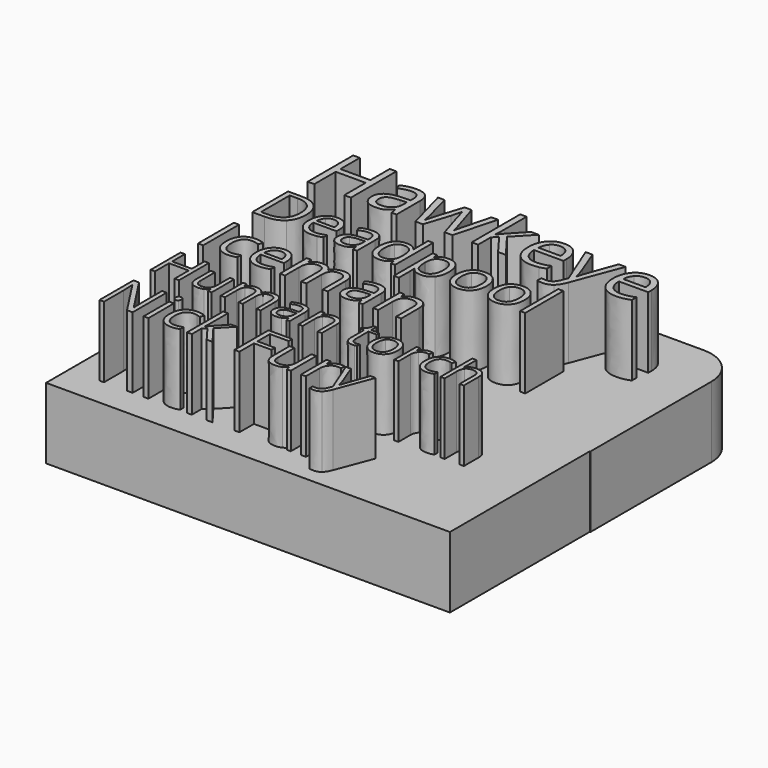
from build123d import *

# Parameters (mm, degrees)
F1_DEPTH     = 25.4
F3_DEPTH     = 25.4
F4_DEPTH     = 25.4
F5_DEPTH     = 25.4
F6_DEPTH     = 25.4
F2_W         = 1.8225440387
F2_H         = 17.0771322931
F7_DEPTH     = 25.4
F2_TEXT_SIZE = 22.4745314982
F8_DEPTH     = 25.4
F9_DEPTH     = 25.4
F10_DEPTH    = 25.4
F2_W_2       = 1.7290800267
F2_H_2       = 11.4105955517
F11_DEPTH    = 25.4
F12_DEPTH    = 25.4
F13_R        = 13.5243778387
F14_R        = 13.5128


# Not quite as in the source:
# - Text() gives the source's letters only with a copy of the font that has no kerning and outlines rounded to 1/6400 em; it was checked with that copy


with BuildPart() as f1:
    # F0 (on Top) → F1 (new body)
    with BuildSketch(Plane.XY):
        Polygon((72.1950531006, 67.6310360432), (-72.6100355387, 67.6310360432), (-72.6100355387, 0), (-72.6100355387, -62.6520514488), (71.9875991344, -62.6520514488), (71.9875991344, 0), (72.1950531006, 0), align=None)
    extrude(amount=F1_DEPTH)

    # F2 (on face) → F3 (join)
    with BuildSketch(Plane.XY.offset(25.4)):
        Polygon((-48.0028636327, 40.0392413139), (-45.6361505882, 40.0392413139), (-45.6361505882, 60.4036705045), (-48.0028636327, 60.4036705045), (-48.0028636327, 51.7390939349), (-58.7310713502, 51.7390939349), (-58.7310713502, 60.4036705045), (-61.0977843947, 60.4036705045), (-61.0977843947, 40.0392413139), (-58.7310713502, 40.0392413139), (-58.7310713502, 49.6219777463), (-48.0028636327, 49.6219777463), align=None)
        with BuildLine():
            Line((-31.4715290151, 42.2142996298), (-31.0124490837, 40.0392413139))
            Line((-31.0124490837, 40.0392413139), (-29.2964706993, 40.0392413139))
            Line((-29.2964706993, 40.0392413139), (-29.2964706993, 50.4599100483))
            add(Edge.make_bspline(
                [(-30.6135398229, 54.3442611185), (-29.2964706993, 53.134162076), (-29.2964706993, 50.4599100483)],
                knots=[0, 0, 0, 1, 1, 1], degree=2))
            add(Edge.make_bspline(
                [(-34.6583460147, 55.554360161), (-31.9306089465, 55.554360161), (-30.6135398229, 54.3442611185)],
                knots=[0, 0, 0, 1, 1, 1], degree=2))
            add(Edge.make_bspline(
                [(-37.3571120193, 55.2067073974), (-36.0133003754, 55.554360161), (-34.6583460147, 55.554360161)],
                knots=[0, 0, 0, 1, 1, 1], degree=2))
            add(Edge.make_bspline(
                [(-39.8285666015, 54.2484337542), (-38.7009236632, 54.8590546338), (-37.3571120193, 55.2067073974)],
                knots=[0, 0, 0, 1, 1, 1], degree=2))
            Line((-39.8285666015, 54.2484337542), (-39.1154327275, 52.4789703292))
            add(Edge.make_bspline(
                [(-34.8009727895, 53.6467270479), (-36.7086059026, 53.6467270479), (-39.1154327275, 52.4789703292)],
                knots=[0, 0, 0, 1, 1, 1], degree=2))
            add(Edge.make_bspline(
                [(-32.327289664, 52.7909663991), (-33.0983656653, 53.6467270479), (-34.8009727895, 53.6467270479)],
                knots=[0, 0, 0, 1, 1, 1], degree=2))
            add(Edge.make_bspline(
                [(-31.5562136626, 50.138999805), (-31.5562136626, 51.9352057502), (-32.327289664, 52.7909663991)],
                knots=[0, 0, 0, 1, 1, 1], degree=2))
            Line((-31.5562136626, 50.138999805), (-31.5562136626, 49.1896403352))
            Line((-31.5562136626, 49.1896403352), (-34.1457810428, 49.1049556877))
            add(Edge.make_bspline(
                [(-41.5400878992, 44.2601024309), (-41.5400878992, 48.882101352), (-34.1457810428, 49.1049556877)],
                knots=[0, 0, 0, 1, 1, 1], degree=2))
            add(Edge.make_bspline(
                [(-40.2519898392, 40.9306586565), (-41.5400878992, 42.1028724619), (-41.5400878992, 44.2601024309)],
                knots=[0, 0, 0, 1, 1, 1], degree=2))
            add(Edge.make_bspline(
                [(-36.6952346424, 39.758444851), (-38.9638917792, 39.758444851), (-40.2519898392, 40.9306586565)],
                knots=[0, 0, 0, 1, 1, 1], degree=2))
            add(Edge.make_bspline(
                [(-33.8582989498, 40.2687812796), (-34.9926275182, 39.758444851), (-36.6952346424, 39.758444851)],
                knots=[0, 0, 0, 1, 1, 1], degree=2))
            add(Edge.make_bspline(
                [(-31.5829561829, 42.2142996298), (-32.7239703814, 40.7791177082), (-33.8582989498, 40.2687812796)],
                knots=[0, 0, 0, 1, 1, 1], degree=2))
            Line((-31.5829561829, 42.2142996298), (-31.4715290151, 42.2142996298))
        make_face()
        with BuildLine():
            add(Edge.make_bspline(
                [(-36.236154711, 41.6705350508), (-34.0744676553, 41.6705350508), (-32.8420831793, 42.853891573)],
                knots=[0, 0, 0, 1, 1, 1], degree=2))
            add(Edge.make_bspline(
                [(-38.3577279863, 42.3234982542), (-37.6000232451, 41.6705350508), (-36.236154711, 41.6705350508)],
                knots=[0, 0, 0, 1, 1, 1], degree=2))
            add(Edge.make_bspline(
                [(-39.1154327275, 44.2333599106), (-39.1154327275, 42.9764614576), (-38.3577279863, 42.3234982542)],
                knots=[0, 0, 0, 1, 1, 1], degree=2))
            add(Edge.make_bspline(
                [(-37.8986480549, 46.593387325), (-39.1154327275, 45.8334540405), (-39.1154327275, 44.2333599106)],
                knots=[0, 0, 0, 1, 1, 1], degree=2))
            add(Edge.make_bspline(
                [(-33.9229267071, 47.4513765172), (-36.6818633823, 47.3533206095), (-37.8986480549, 46.593387325)],
                knots=[0, 0, 0, 1, 1, 1], degree=2))
            Line((-33.9229267071, 47.4513765172), (-31.6096987032, 47.5449753382))
            Line((-31.6096987032, 47.5449753382), (-31.6096987032, 46.167735544))
            add(Edge.make_bspline(
                [(-32.8420831793, 42.853891573), (-31.6096987032, 44.0372480953), (-31.6096987032, 46.167735544)],
                knots=[0, 0, 0, 1, 1, 1], degree=2))
        make_face(mode=Mode.SUBTRACT)
        with BuildLine():
            Line((-14.8688810101, 48.9935285198), (-12.0698305545, 40.0392413139))
            Line((-12.0698305545, 40.0392413139), (-9.3242651395, 40.0392413139))
            Line((-9.3242651395, 40.0392413139), (-5.1078611092, 55.3047633051))
            Line((-5.1078611092, 55.3047633051), (-7.501316674, 55.3047633051))
            add(Edge.make_bspline(
                [(-10.4051086673, 44.0662191589), (-10.1621974415, 45.111405993), (-7.501316674, 55.3047633051)],
                knots=[0, 0, 0, 1, 1, 1], degree=2))
            add(Edge.make_bspline(
                [(-10.7059620204, 42.5173815262), (-10.6480198932, 43.0210323248), (-10.4051086673, 44.0662191589)],
                knots=[0, 0, 0, 1, 1, 1], degree=2))
            Line((-10.7059620204, 42.5173815262), (-10.8173891883, 42.5173815262))
            add(Edge.make_bspline(
                [(-11.8737187392, 46.5421308278), (-11.0937285644, 44.1486752631), (-10.8173891883, 42.5173815262)],
                knots=[0, 0, 0, 1, 1, 1], degree=2))
            Line((-11.8737187392, 46.5421308278), (-14.6059128941, 55.3047633051))
            Line((-14.6059128941, 55.3047633051), (-17.1107956266, 55.3047633051))
            Line((-17.1107956266, 55.3047633051), (-19.9098460823, 46.5421308278))
            add(Edge.make_bspline(
                [(-20.5048671584, 44.5453559805), (-20.1639000249, 45.8067115202), (-19.9098460823, 46.5421308278)],
                knots=[0, 0, 0, 1, 1, 1], degree=2))
            add(Edge.make_bspline(
                [(-20.9973752402, 42.4906390059), (-20.8458342919, 43.2840004408), (-20.5048671584, 44.5453559805)],
                knots=[0, 0, 0, 1, 1, 1], degree=2))
            Line((-20.9973752402, 42.4906390059), (-21.108802408, 42.4906390059))
            add(Edge.make_bspline(
                [(-21.9935341205, 46.5421308278), (-21.2202295758, 43.5335972967), (-21.108802408, 42.4906390059)],
                knots=[0, 0, 0, 1, 1, 1], degree=2))
            add(Edge.make_bspline(
                [(-24.242134367, 55.3047633051), (-22.7668386651, 49.5506643589), (-21.9935341205, 46.5421308278)],
                knots=[0, 0, 0, 1, 1, 1], degree=2))
            Line((-24.242134367, 55.3047633051), (-26.6667895388, 55.3047633051))
            Line((-26.6667895388, 55.3047633051), (-22.5038705491, 40.0392413139))
            Line((-22.5038705491, 40.0392413139), (-19.8296185214, 40.0392413139))
            Line((-19.8296185214, 40.0392413139), (-16.9458834183, 48.9667859996))
            add(Edge.make_bspline(
                [(-15.9697814282, 52.7285671851), (-16.5269172673, 50.2905407532), (-16.9458834183, 48.9667859996)],
                knots=[0, 0, 0, 1, 1, 1], degree=2))
            Line((-15.9697814282, 52.7285671851), (-15.8583542604, 52.7285671851))
            add(Edge.make_bspline(
                [(-14.8688810101, 48.9935285198), (-15.1363062129, 49.8180895617), (-15.8583542604, 52.7285671851)],
                knots=[0, 0, 0, 1, 1, 1], degree=2))
        make_face()
    extrude(amount=F3_DEPTH)

    # F2 (on face) → F4 (join)
    with BuildSketch(Plane.XY.offset(25.4)):
        with BuildLine():
            add(Edge.make_bspline(
                [(-0.0624389504, 47.8525143214), (0.5348106691, 48.7038178835), (1.7605095151, 50.0810576777)],
                knots=[0, 0, 0, 1, 1, 1], degree=2))
            Line((-0.0624389504, 47.8525143214), (-0.1738661182, 47.8525143214))
            add(Edge.make_bspline(
                [(-0.0624389504, 50.2192273658), (-0.0624389504, 49.457065538), (-0.1738661182, 47.8525143214)],
                knots=[0, 0, 0, 1, 1, 1], degree=2))
            Line((-0.0624389504, 50.2192273658), (-0.0624389504, 61.714053998))
            Line((-0.0624389504, 61.714053998), (-2.348924434, 61.714053998))
            Line((-2.348924434, 61.714053998), (-2.348924434, 40.0392413139))
            Line((-2.348924434, 40.0392413139), (-0.0624389504, 40.0392413139))
            Line((-0.0624389504, 40.0392413139), (-0.0624389504, 45.748769393))
            Line((-0.0624389504, 45.748769393), (1.6758248676, 47.2552647019))
            Line((1.6758248676, 47.2552647019), (7.06889979, 40.0392413139))
            Line((7.06889979, 40.0392413139), (9.8679502456, 40.0392413139))
            Line((9.8679502456, 40.0392413139), (3.2491764772, 48.8018737912))
            Line((3.2491764772, 48.8018737912), (9.4356128344, 55.3047633051))
            Line((9.4356128344, 55.3047633051), (6.6900474194, 55.3047633051))
            Line((6.6900474194, 55.3047633051), (1.7605095151, 50.0810576777))
        make_face()
        with BuildLine():
            add(Edge.make_bspline(
                [(19.0718343074, 39.758444851), (15.6889054924, 39.758444851), (13.7300158822, 41.822075999)],
                knots=[0, 0, 0, 1, 1, 1], degree=2))
            add(Edge.make_bspline(
                [(21.7104296413, 39.9902133601), (20.6184433967, 39.758444851), (19.0718343074, 39.758444851)],
                knots=[0, 0, 0, 1, 1, 1], degree=2))
            add(Edge.make_bspline(
                [(24.028114732, 40.7479181013), (22.802415886, 40.2219818692), (21.7104296413, 39.9902133601)],
                knots=[0, 0, 0, 1, 1, 1], degree=2))
            Line((24.028114732, 40.7479181013), (24.028114732, 42.8115492493))
            add(Edge.make_bspline(
                [(19.1565189549, 41.7819622186), (21.6212879071, 41.7819622186), (24.028114732, 42.8115492493)],
                knots=[0, 0, 0, 1, 1, 1], degree=2))
            add(Edge.make_bspline(
                [(15.5284503708, 43.1748018163), (16.8165484307, 41.7819622186), (19.1565189549, 41.7819622186)],
                knots=[0, 0, 0, 1, 1, 1], degree=2))
            add(Edge.make_bspline(
                [(14.1690389234, 47.2552647019), (14.2403523108, 44.5676414141), (15.5284503708, 43.1748018163)],
                knots=[0, 0, 0, 1, 1, 1], degree=2))
            Line((14.1690389234, 47.2552647019), (24.6833064787, 47.2552647019))
            Line((24.6833064787, 47.2552647019), (24.6833064787, 48.7171891436))
            add(Edge.make_bspline(
                [(23.0118989615, 53.6979835451), (24.6833064787, 51.8104073223), (24.6833064787, 48.7171891436)],
                knots=[0, 0, 0, 1, 1, 1], degree=2))
            add(Edge.make_bspline(
                [(18.4745846879, 55.585559768), (21.3404914442, 55.585559768), (23.0118989615, 53.6979835451)],
                knots=[0, 0, 0, 1, 1, 1], degree=2))
            add(Edge.make_bspline(
                [(13.5896176507, 53.4127299955), (15.4081090295, 55.585559768), (18.4745846879, 55.585559768)],
                knots=[0, 0, 0, 1, 1, 1], degree=2))
            add(Edge.make_bspline(
                [(11.7711262719, 47.5449753382), (11.7711262719, 51.2399002231), (13.5896176507, 53.4127299955)],
                knots=[0, 0, 0, 1, 1, 1], degree=2))
            add(Edge.make_bspline(
                [(13.7300158822, 41.822075999), (11.7711262719, 43.885707147), (11.7711262719, 47.5449753382)],
                knots=[0, 0, 0, 1, 1, 1], degree=2))
        make_face()
        with BuildLine():
            add(Edge.make_bspline(
                [(18.4433850809, 53.6467270479), (16.6070653552, 53.6467270479), (15.5128505673, 52.4499992656)],
                knots=[0, 0, 0, 1, 1, 1], degree=2))
            add(Edge.make_bspline(
                [(21.2312928197, 52.4834274159), (20.257419373, 53.6467270479), (18.4433850809, 53.6467270479)],
                knots=[0, 0, 0, 1, 1, 1], degree=2))
            add(Edge.make_bspline(
                [(22.2051662665, 49.1361552946), (22.2051662665, 51.3201277839), (21.2312928197, 52.4834274159)],
                knots=[0, 0, 0, 1, 1, 1], degree=2))
            Line((22.2051662665, 49.1361552946), (14.2225239639, 49.1361552946))
            add(Edge.make_bspline(
                [(15.5128505673, 52.4499992656), (14.4186357793, 51.2532714832), (14.2225239639, 49.1361552946)],
                knots=[0, 0, 0, 1, 1, 1], degree=2))
        make_face(mode=Mode.SUBTRACT)
        with BuildLine():
            Line((28.6857703468, 55.3047633051), (26.2031730478, 55.3047633051))
            Line((26.2031730478, 55.3047633051), (32.3628668848, 39.9545566664))
            Line((32.3628668848, 39.9545566664), (31.5115633227, 37.7839554373))
            add(Edge.make_bspline(
                [(28.1108061608, 35.1097034096), (30.4953475522, 35.1097034096), (31.5115633227, 37.7839554373)],
                knots=[0, 0, 0, 1, 1, 1], degree=2))
            add(Edge.make_bspline(
                [(26.3992848631, 35.274615618), (27.1659037777, 35.1097034096), (28.1108061608, 35.1097034096)],
                knots=[0, 0, 0, 1, 1, 1], degree=2))
            Line((26.3992848631, 35.274615618), (26.3992848631, 33.4249246322))
            add(Edge.make_bspline(
                [(28.4896585314, 33.1842419497), (27.4288718938, 33.1842419497), (26.3992848631, 33.4249246322)],
                knots=[0, 0, 0, 1, 1, 1], degree=2))
            add(Edge.make_bspline(
                [(31.6853897045, 34.2650854776), (30.3839203843, 33.1842419497), (28.4896585314, 33.1842419497)],
                knots=[0, 0, 0, 1, 1, 1], degree=2))
            add(Edge.make_bspline(
                [(33.9629610147, 37.9221251254), (32.9868590246, 35.3459290054), (31.6853897045, 34.2650854776)],
                knots=[0, 0, 0, 1, 1, 1], degree=2))
            Line((33.9629610147, 37.9221251254), (40.5237926558, 55.3047633051))
            Line((40.5237926558, 55.3047633051), (38.0456524435, 55.3047633051))
            add(Edge.make_bspline(
                [(34.2615858244, 44.7280965357), (34.8410070971, 46.4485320069), (38.0456524435, 55.3047633051)],
                knots=[0, 0, 0, 1, 1, 1], degree=2))
            add(Edge.make_bspline(
                [(33.5038810833, 42.2945271906), (33.6821645518, 43.0076610646), (34.2615858244, 44.7280965357)],
                knots=[0, 0, 0, 1, 1, 1], degree=2))
            Line((33.5038810833, 42.2945271906), (33.3924539154, 42.2945271906))
            add(Edge.make_bspline(
                [(32.0285853813, 46.6000729551), (33.1250287127, 43.6182819443), (33.3924539154, 42.2945271906)],
                knots=[0, 0, 0, 1, 1, 1], degree=2))
            Line((32.0285853813, 46.6000729551), (28.6857703468, 55.3047633051))
        make_face()
    extrude(amount=F4_DEPTH)

    # F2 (on face) → F5 (join)
    with BuildSketch(Plane.XY.offset(25.4)):
        with BuildLine():
            add(Edge.make_bspline(
                [(49.4513373415, 39.758444851), (46.0684085265, 39.758444851), (44.1095189162, 41.822075999)],
                knots=[0, 0, 0, 1, 1, 1], degree=2))
            add(Edge.make_bspline(
                [(52.0899326754, 39.9902133601), (50.9979464308, 39.758444851), (49.4513373415, 39.758444851)],
                knots=[0, 0, 0, 1, 1, 1], degree=2))
            add(Edge.make_bspline(
                [(54.407617766, 40.7479181013), (53.18191892, 40.2219818692), (52.0899326754, 39.9902133601)],
                knots=[0, 0, 0, 1, 1, 1], degree=2))
            Line((54.407617766, 40.7479181013), (54.407617766, 42.8115492493))
            add(Edge.make_bspline(
                [(49.536021989, 41.7819622186), (52.0007909411, 41.7819622186), (54.407617766, 42.8115492493)],
                knots=[0, 0, 0, 1, 1, 1], degree=2))
            add(Edge.make_bspline(
                [(45.9079534048, 43.1748018163), (47.1960514648, 41.7819622186), (49.536021989, 41.7819622186)],
                knots=[0, 0, 0, 1, 1, 1], degree=2))
            add(Edge.make_bspline(
                [(44.5485419574, 47.2552647019), (44.6198553448, 44.5676414141), (45.9079534048, 43.1748018163)],
                knots=[0, 0, 0, 1, 1, 1], degree=2))
            Line((44.5485419574, 47.2552647019), (55.0628095128, 47.2552647019))
            Line((55.0628095128, 47.2552647019), (55.0628095128, 48.7171891436))
            add(Edge.make_bspline(
                [(53.3914019955, 53.6979835451), (55.0628095128, 51.8104073223), (55.0628095128, 48.7171891436)],
                knots=[0, 0, 0, 1, 1, 1], degree=2))
            add(Edge.make_bspline(
                [(48.8540877219, 55.585559768), (51.7199944782, 55.585559768), (53.3914019955, 53.6979835451)],
                knots=[0, 0, 0, 1, 1, 1], degree=2))
            add(Edge.make_bspline(
                [(43.9691206848, 53.4127299955), (45.7876120636, 55.585559768), (48.8540877219, 55.585559768)],
                knots=[0, 0, 0, 1, 1, 1], degree=2))
            add(Edge.make_bspline(
                [(42.150629306, 47.5449753382), (42.150629306, 51.2399002231), (43.9691206848, 53.4127299955)],
                knots=[0, 0, 0, 1, 1, 1], degree=2))
            add(Edge.make_bspline(
                [(44.1095189162, 41.822075999), (42.150629306, 43.885707147), (42.150629306, 47.5449753382)],
                knots=[0, 0, 0, 1, 1, 1], degree=2))
        make_face()
        with BuildLine():
            add(Edge.make_bspline(
                [(48.822888115, 53.6467270479), (46.9865683893, 53.6467270479), (45.8923536013, 52.4499992656)],
                knots=[0, 0, 0, 1, 1, 1], degree=2))
            add(Edge.make_bspline(
                [(51.6107958538, 52.4834274159), (50.636922407, 53.6467270479), (48.822888115, 53.6467270479)],
                knots=[0, 0, 0, 1, 1, 1], degree=2))
            add(Edge.make_bspline(
                [(52.5846693005, 49.1361552946), (52.5846693005, 51.3201277839), (51.6107958538, 52.4834274159)],
                knots=[0, 0, 0, 1, 1, 1], degree=2))
            Line((52.5846693005, 49.1361552946), (44.602026998, 49.1361552946))
            add(Edge.make_bspline(
                [(45.8923536013, 52.4499992656), (44.7981388133, 51.2532714832), (44.602026998, 49.1361552946)],
                knots=[0, 0, 0, 1, 1, 1], degree=2))
        make_face(mode=Mode.SUBTRACT)
    extrude(amount=F5_DEPTH)

    # F2 (on face) → F6 (join)
    with BuildSketch(Plane.XY.offset(25.4)):
        with BuildLine():
            add(Edge.make_bspline(
                [(-48.8845501386, 24.1493195451), (-48.8845501386, 20.1776484319), (-51.0407005042, 18.0759285722)],
                knots=[0, 0, 0, 1, 1, 1], degree=2))
            add(Edge.make_bspline(
                [(-50.9581768339, 29.9452905197), (-48.8845501386, 27.8716638244), (-48.8845501386, 24.1493195451)],
                knots=[0, 0, 0, 1, 1, 1], degree=2))
            add(Edge.make_bspline(
                [(-56.7752176818, 32.018917215), (-53.0318035291, 32.018917215), (-50.9581768339, 29.9452905197)],
                knots=[0, 0, 0, 1, 1, 1], degree=2))
            Line((-56.7752176818, 32.018917215), (-61.691521447, 32.018917215))
            Line((-61.691521447, 32.018917215), (-61.691521447, 15.9742087126))
            Line((-61.691521447, 15.9742087126), (-57.2457781851, 15.9742087126))
            add(Edge.make_bspline(
                [(-51.0407005042, 18.0759285722), (-53.1968508698, 15.9742087126), (-57.2457781851, 15.9742087126)],
                knots=[0, 0, 0, 1, 1, 1], degree=2))
        make_face()
        with BuildLine():
            add(Edge.make_bspline(
                [(-50.8580949358, 24.0825982797), (-50.8580949358, 27.2220093983), (-52.4330679634, 28.8127848309)],
                knots=[0, 0, 0, 1, 1, 1], degree=2))
            add(Edge.make_bspline(
                [(-52.5384173298, 19.2277483115), (-50.8580949358, 20.8694426045), (-50.8580949358, 24.0825982797)],
                knots=[0, 0, 0, 1, 1, 1], degree=2))
            add(Edge.make_bspline(
                [(-57.5548029932, 17.5860540185), (-54.2187397239, 17.5860540185), (-52.5384173298, 19.2277483115)],
                knots=[0, 0, 0, 1, 1, 1], degree=2))
            Line((-57.5548029932, 17.5860540185), (-59.8268376618, 17.5860540185))
            Line((-59.8268376618, 17.5860540185), (-59.8268376618, 30.4035602635))
            Line((-59.8268376618, 30.4035602635), (-57.1158472998, 30.4035602635))
            add(Edge.make_bspline(
                [(-52.4330679634, 28.8127848309), (-54.0080409911, 30.4035602635), (-57.1158472998, 30.4035602635)],
                knots=[0, 0, 0, 1, 1, 1], degree=2))
        make_face(mode=Mode.SUBTRACT)
        with BuildLine():
            add(Edge.make_bspline(
                [(-40.4987405733, 15.7529750431), (-43.1640795432, 15.7529750431), (-44.7074477609, 17.3788669312)],
                knots=[0, 0, 0, 1, 1, 1], degree=2))
            add(Edge.make_bspline(
                [(-38.4198464098, 15.9355806116), (-39.2801995687, 15.7529750431), (-40.4987405733, 15.7529750431)],
                knots=[0, 0, 0, 1, 1, 1], degree=2))
            add(Edge.make_bspline(
                [(-36.5937907255, 16.5325603545), (-37.5594932508, 16.11818618), (-38.4198464098, 15.9355806116)],
                knots=[0, 0, 0, 1, 1, 1], degree=2))
            Line((-36.5937907255, 16.5325603545), (-36.5937907255, 18.1584522426))
            add(Edge.make_bspline(
                [(-40.432019308, 17.3472621213), (-38.4900793207, 17.3472621213), (-36.5937907255, 18.1584522426)],
                knots=[0, 0, 0, 1, 1, 1], degree=2))
            add(Edge.make_bspline(
                [(-43.2904987829, 18.4446513546), (-42.2756332199, 17.3472621213), (-40.432019308, 17.3472621213)],
                knots=[0, 0, 0, 1, 1, 1], degree=2))
            add(Edge.make_bspline(
                [(-44.3615506746, 21.6595628525), (-44.3053643458, 19.5420405879), (-43.2904987829, 18.4446513546)],
                knots=[0, 0, 0, 1, 1, 1], degree=2))
            Line((-44.3615506746, 21.6595628525), (-36.0775788302, 21.6595628525))
            Line((-36.0775788302, 21.6595628525), (-36.0775788302, 22.8113825918))
            add(Edge.make_bspline(
                [(-37.3944459101, 26.7356464901), (-36.0775788302, 25.2484646011), (-36.0775788302, 22.8113825918)],
                knots=[0, 0, 0, 1, 1, 1], degree=2))
            add(Edge.make_bspline(
                [(-40.9693010766, 28.2228283791), (-38.7113129901, 28.2228283791), (-37.3944459101, 26.7356464901)],
                knots=[0, 0, 0, 1, 1, 1], degree=2))
            add(Edge.make_bspline(
                [(-44.8180645957, 26.5109011751), (-43.3853132126, 28.2228283791), (-40.9693010766, 28.2228283791)],
                knots=[0, 0, 0, 1, 1, 1], degree=2))
            add(Edge.make_bspline(
                [(-46.2508159787, 21.887819813), (-46.2508159787, 24.7989739712), (-44.8180645957, 26.5109011751)],
                knots=[0, 0, 0, 1, 1, 1], degree=2))
            add(Edge.make_bspline(
                [(-44.7074477609, 17.3788669312), (-46.2508159787, 19.0047588193), (-46.2508159787, 21.887819813)],
                knots=[0, 0, 0, 1, 1, 1], degree=2))
        make_face()
        with BuildLine():
            add(Edge.make_bspline(
                [(-40.9938825954, 26.6952625663), (-42.4406805606, 26.6952625663), (-43.3027895423, 25.7523857371)],
                knots=[0, 0, 0, 1, 1, 1], degree=2))
            add(Edge.make_bspline(
                [(-38.797348306, 25.7787230787), (-39.5646428579, 26.6952625663), (-40.9938825954, 26.6952625663)],
                knots=[0, 0, 0, 1, 1, 1], degree=2))
            add(Edge.make_bspline(
                [(-38.0300537541, 23.1414772732), (-38.0300537541, 24.862183591), (-38.797348306, 25.7787230787)],
                knots=[0, 0, 0, 1, 1, 1], degree=2))
            Line((-38.0300537541, 23.1414772732), (-44.319410928, 23.1414772732))
            add(Edge.make_bspline(
                [(-43.3027895423, 25.7523857371), (-44.164898524, 24.8095089078), (-44.319410928, 23.1414772732)],
                knots=[0, 0, 0, 1, 1, 1], degree=2))
        make_face(mode=Mode.SUBTRACT)
        with BuildLine():
            Line((-25.9359464916, 17.6878917393), (-25.5742470003, 15.9742087126))
            Line((-25.5742470003, 15.9742087126), (-24.2222634649, 15.9742087126))
            Line((-24.2222634649, 15.9742087126), (-24.2222634649, 24.1844360005))
            add(Edge.make_bspline(
                [(-25.2599547239, 27.2448350944), (-24.2222634649, 26.2914233285), (-24.2222634649, 24.1844360005)],
                knots=[0, 0, 0, 1, 1, 1], degree=2))
            add(Edge.make_bspline(
                [(-28.4467730574, 28.1982468603), (-26.2976459829, 28.1982468603), (-25.2599547239, 27.2448350944)],
                knots=[0, 0, 0, 1, 1, 1], degree=2))
            add(Edge.make_bspline(
                [(-30.5730744359, 27.9243385076), (-29.5143133036, 28.1982468603), (-28.4467730574, 28.1982468603)],
                knots=[0, 0, 0, 1, 1, 1], degree=2))
            add(Edge.make_bspline(
                [(-32.5202818915, 27.1693347151), (-31.6318355682, 27.650430155), (-30.5730744359, 27.9243385076)],
                knots=[0, 0, 0, 1, 1, 1], degree=2))
            Line((-32.5202818915, 27.1693347151), (-31.958418604, 25.7752114331))
            add(Edge.make_bspline(
                [(-28.5591457149, 26.6952625663), (-30.0621300089, 26.6952625663), (-31.958418604, 25.7752114331)],
                knots=[0, 0, 0, 1, 1, 1], degree=2))
            add(Edge.make_bspline(
                [(-26.6101824365, 26.0210266214), (-27.2176971161, 26.6952625663), (-28.5591457149, 26.6952625663)],
                knots=[0, 0, 0, 1, 1, 1], degree=2))
            add(Edge.make_bspline(
                [(-26.002667757, 23.9315975212), (-26.002667757, 25.3467906764), (-26.6101824365, 26.0210266214)],
                knots=[0, 0, 0, 1, 1, 1], degree=2))
            Line((-26.002667757, 23.9315975212), (-26.002667757, 23.1836170197))
            Line((-26.002667757, 23.1836170197), (-28.0429338196, 23.1168957544))
            add(Edge.make_bspline(
                [(-33.8687537814, 19.2997370452), (-33.8687537814, 22.941313477), (-28.0429338196, 23.1168957544)],
                knots=[0, 0, 0, 1, 1, 1], degree=2))
            add(Edge.make_bspline(
                [(-32.8538882184, 16.6765378219), (-33.8687537814, 17.6001006007), (-33.8687537814, 19.2997370452)],
                knots=[0, 0, 0, 1, 1, 1], degree=2))
            add(Edge.make_bspline(
                [(-30.0515950722, 15.7529750431), (-31.8390226554, 15.7529750431), (-32.8538882184, 16.6765378219)],
                knots=[0, 0, 0, 1, 1, 1], degree=2))
            add(Edge.make_bspline(
                [(-27.8164326818, 16.1550584582), (-28.7101464734, 15.7529750431), (-30.0515950722, 15.7529750431)],
                knots=[0, 0, 0, 1, 1, 1], degree=2))
            add(Edge.make_bspline(
                [(-26.0237376303, 17.6878917393), (-26.9227188902, 16.5571418733), (-27.8164326818, 16.1550584582)],
                knots=[0, 0, 0, 1, 1, 1], degree=2))
            Line((-26.0237376303, 17.6878917393), (-25.9359464916, 17.6878917393))
        make_face()
        with BuildLine():
            add(Edge.make_bspline(
                [(-29.6898955809, 17.2594709826), (-27.9867474908, 17.2594709826), (-27.0157774972, 18.1918128753)],
                knots=[0, 0, 0, 1, 1, 1], degree=2))
            add(Edge.make_bspline(
                [(-31.3614388611, 17.7739270552), (-30.7644591182, 17.2594709826), (-29.6898955809, 17.2594709826)],
                knots=[0, 0, 0, 1, 1, 1], degree=2))
            add(Edge.make_bspline(
                [(-31.958418604, 19.2786671719), (-31.958418604, 18.2883831278), (-31.3614388611, 17.7739270552)],
                knots=[0, 0, 0, 1, 1, 1], degree=2))
            add(Edge.make_bspline(
                [(-30.9997393698, 21.1380834888), (-31.958418604, 20.5393479232), (-31.958418604, 19.2786671719)],
                knots=[0, 0, 0, 1, 1, 1], degree=2))
            add(Edge.make_bspline(
                [(-27.8673515422, 21.8140752566), (-30.0410601356, 21.7368190545), (-30.9997393698, 21.1380834888)],
                knots=[0, 0, 0, 1, 1, 1], degree=2))
            Line((-27.8673515422, 21.8140752566), (-26.0448075035, 21.887819813))
            Line((-26.0448075035, 21.887819813), (-26.0448075035, 20.8027213391))
            add(Edge.make_bspline(
                [(-27.0157774972, 18.1918128753), (-26.0448075035, 19.1241547679), (-26.0448075035, 20.8027213391)],
                knots=[0, 0, 0, 1, 1, 1], degree=2))
        make_face(mode=Mode.SUBTRACT)
        with BuildLine():
            Line((-12.3845063273, 17.5860540185), (-12.286180252, 17.5860540185))
            Line((-12.286180252, 17.5860540185), (-12.0438767093, 15.9742087126))
            Line((-12.0438767093, 15.9742087126), (-10.5619622886, 15.9742087126))
            Line((-10.5619622886, 15.9742087126), (-10.5619622886, 33.0513410057))
            Line((-10.5619622886, 33.0513410057), (-12.3845063273, 33.0513410057))
            Line((-12.3845063273, 33.0513410057), (-12.3845063273, 28.1561071137))
            Line((-12.3845063273, 28.1561071137), (-12.3388549352, 27.309800537))
            Line((-12.3388549352, 27.309800537), (-12.2615987332, 26.442424087))
            Line((-12.2615987332, 26.442424087), (-12.4055762006, 26.442424087))
            add(Edge.make_bspline(
                [(-16.1595252899, 28.2228283791), (-13.7119083439, 28.2228283791), (-12.4055762006, 26.442424087)],
                knots=[0, 0, 0, 1, 1, 1], degree=2))
            add(Edge.make_bspline(
                [(-19.8256832405, 26.5758666178), (-18.5088161605, 28.2228283791), (-16.1595252899, 28.2228283791)],
                knots=[0, 0, 0, 1, 1, 1], degree=2))
            add(Edge.make_bspline(
                [(-21.1425503205, 21.9545410784), (-21.1425503205, 24.9289048564), (-19.8256832405, 26.5758666178)],
                knots=[0, 0, 0, 1, 1, 1], degree=2))
            add(Edge.make_bspline(
                [(-19.8309507088, 17.3665761718), (-21.1425503205, 18.9801773005), (-21.1425503205, 21.9545410784)],
                knots=[0, 0, 0, 1, 1, 1], degree=2))
            add(Edge.make_bspline(
                [(-16.1595252899, 15.7529750431), (-18.5193510972, 15.7529750431), (-19.8309507088, 17.3665761718)],
                knots=[0, 0, 0, 1, 1, 1], degree=2))
            add(Edge.make_bspline(
                [(-12.3845063273, 17.5860540185), (-13.6451870785, 15.7529750431), (-16.1595252899, 15.7529750431)],
                knots=[0, 0, 0, 1, 1, 1], degree=2))
        make_face()
        with BuildLine():
            add(Edge.make_bspline(
                [(-15.9277566838, 17.2805408559), (-14.0630728986, 17.2805408559), (-13.2237896129, 18.2954064189)],
                knots=[0, 0, 0, 1, 1, 1], degree=2))
            add(Edge.make_bspline(
                [(-18.4087342625, 18.4551862912), (-17.5641835085, 17.2805408559), (-15.9277566838, 17.2805408559)],
                knots=[0, 0, 0, 1, 1, 1], degree=2))
            add(Edge.make_bspline(
                [(-19.2532850164, 21.9334712052), (-19.2532850164, 19.6298317266), (-18.4087342625, 18.4551862912)],
                knots=[0, 0, 0, 1, 1, 1], degree=2))
            add(Edge.make_bspline(
                [(-18.4034667941, 25.4503842201), (-19.2532850164, 24.2055058738), (-19.2532850164, 21.9334712052)],
                knots=[0, 0, 0, 1, 1, 1], degree=2))
            add(Edge.make_bspline(
                [(-15.9488265571, 26.6952625663), (-17.5536485719, 26.6952625663), (-18.4034667941, 25.4503842201)],
                knots=[0, 0, 0, 1, 1, 1], degree=2))
            add(Edge.make_bspline(
                [(-13.2343245496, 25.6031408013), (-14.0841427718, 26.6952625663), (-15.9488265571, 26.6952625663)],
                knots=[0, 0, 0, 1, 1, 1], degree=2))
            add(Edge.make_bspline(
                [(-12.3845063273, 21.9545410784), (-12.3845063273, 24.5110190364), (-13.2343245496, 25.6031408013)],
                knots=[0, 0, 0, 1, 1, 1], degree=2))
            Line((-12.3845063273, 21.9545410784), (-12.3845063273, 21.5717717139))
            add(Edge.make_bspline(
                [(-13.2237896129, 18.2954064189), (-12.3845063273, 19.3102719818), (-12.3845063273, 21.5717717139)],
                knots=[0, 0, 0, 1, 1, 1], degree=2))
        make_face(mode=Mode.SUBTRACT)
        with BuildLine():
            add(Edge.make_bspline(
                [(-1.1015891861, 15.7529750431), (-2.2779904442, 15.7529750431), (-3.2489604378, 16.1866632681)],
                knots=[0, 0, 0, 1, 1, 1], degree=2))
            add(Edge.make_bspline(
                [(2.5698362329, 17.3946693362), (1.2477016846, 15.7529750431), (-1.1015891861, 15.7529750431)],
                knots=[0, 0, 0, 1, 1, 1], degree=2))
            add(Edge.make_bspline(
                [(3.8919707812, 22.0001924705), (3.8919707812, 19.0363636292), (2.5698362329, 17.3946693362)],
                knots=[0, 0, 0, 1, 1, 1], degree=2))
            add(Edge.make_bspline(
                [(2.5909061062, 26.5864015544), (3.8919707812, 24.9499747297), (3.8919707812, 22.0001924705)],
                knots=[0, 0, 0, 1, 1, 1], degree=2))
            add(Edge.make_bspline(
                [(-1.1015891861, 28.2228283791), (1.2898414312, 28.2228283791), (2.5909061062, 26.5864015544)],
                knots=[0, 0, 0, 1, 1, 1], degree=2))
            add(Edge.make_bspline(
                [(-3.2419371467, 27.7838726858), (-2.3095952541, 28.2228283791), (-1.1015891861, 28.2228283791)],
                knots=[0, 0, 0, 1, 1, 1], degree=2))
            add(Edge.make_bspline(
                [(-4.8766081487, 26.3546329483), (-4.1742790393, 27.3449169925), (-3.2419371467, 27.7838726858)],
                knots=[0, 0, 0, 1, 1, 1], degree=2))
            Line((-4.8766081487, 26.3546329483), (-4.9643992873, 26.3546329483))
            Line((-4.9643992873, 26.3546329483), (-5.2172377667, 28.0015947097))
            Line((-5.2172377667, 28.0015947097), (-6.6991521873, 28.0015947097))
            Line((-6.6991521873, 28.0015947097), (-6.6991521873, 10.5732978619))
            Line((-6.6991521873, 10.5732978619), (-4.8766081487, 10.5732978619))
            Line((-4.8766081487, 10.5732978619), (-4.8766081487, 15.5247180826))
            add(Edge.make_bspline(
                [(-5.0100506794, 17.5228443986), (-4.8766081487, 16.4693507346), (-4.8766081487, 15.5247180826)],
                knots=[0, 0, 0, 1, 1, 1], degree=2))
            Line((-5.0100506794, 17.5228443986), (-4.8766081487, 17.5228443986))
            add(Edge.make_bspline(
                [(-3.2489604378, 16.1866632681), (-4.2199304314, 16.6203514932), (-4.8766081487, 17.5228443986)],
                knots=[0, 0, 0, 1, 1, 1], degree=2))
        make_face()
        with BuildLine():
            add(Edge.make_bspline(
                [(-1.3649626021, 26.6741926931), (-3.208576514, 26.6741926931), (-4.0320573947, 25.6540596618)],
                knots=[0, 0, 0, 1, 1, 1], degree=2))
            add(Edge.make_bspline(
                [(1.1195266222, 25.4732099161), (0.2363477672, 26.6741926931), (-1.3649626021, 26.6741926931)],
                knots=[0, 0, 0, 1, 1, 1], degree=2))
            add(Edge.make_bspline(
                [(2.0027054771, 22.0212623438), (2.0027054771, 24.2722271392), (1.1195266222, 25.4732099161)],
                knots=[0, 0, 0, 1, 1, 1], degree=2))
            add(Edge.make_bspline(
                [(1.1195266222, 18.5429774299), (2.0027054771, 19.8054140039), (2.0027054771, 22.0212623438)],
                knots=[0, 0, 0, 1, 1, 1], degree=2))
            add(Edge.make_bspline(
                [(-1.3228228555, 17.2805408559), (0.2363477672, 17.2805408559), (1.1195266222, 18.5429774299)],
                knots=[0, 0, 0, 1, 1, 1], degree=2))
            add(Edge.make_bspline(
                [(-4.0320573947, 18.3726626209), (-3.1875066407, 17.2805408559), (-1.3228228555, 17.2805408559)],
                knots=[0, 0, 0, 1, 1, 1], degree=2))
            add(Edge.make_bspline(
                [(-4.8766081487, 22.0001924705), (-4.8766081487, 19.4647843859), (-4.0320573947, 18.3726626209)],
                knots=[0, 0, 0, 1, 1, 1], degree=2))
            Line((-4.8766081487, 22.0001924705), (-4.8766081487, 22.4040317084))
            add(Edge.make_bspline(
                [(-4.0320573947, 25.6540596618), (-4.8555382754, 24.6339266305), (-4.8766081487, 22.4040317084)],
                knots=[0, 0, 0, 1, 1, 1], degree=2))
        make_face(mode=Mode.SUBTRACT)
        with BuildLine():
            add(Edge.make_bspline(
                [(17.4539458822, 22.0001924705), (17.4539458822, 19.0574335025), (15.9737872843, 17.4052042728)],
                knots=[0, 0, 0, 1, 1, 1], degree=2))
            add(Edge.make_bspline(
                [(15.9667639932, 26.5425059851), (17.4539458822, 24.862183591), (17.4539458822, 22.0001924705)],
                knots=[0, 0, 0, 1, 1, 1], degree=2))
            add(Edge.make_bspline(
                [(11.9582206017, 28.2228283791), (14.4795821042, 28.2228283791), (15.9667639932, 26.5425059851)],
                knots=[0, 0, 0, 1, 1, 1], degree=2))
            add(Edge.make_bspline(
                [(7.874176831, 26.5811340861), (9.3455563151, 28.2228283791), (11.9582206017, 28.2228283791)],
                knots=[0, 0, 0, 1, 1, 1], degree=2))
            add(Edge.make_bspline(
                [(6.402797347, 22.0001924705), (6.402797347, 24.939439793), (7.874176831, 26.5811340861)],
                knots=[0, 0, 0, 1, 1, 1], degree=2))
            add(Edge.make_bspline(
                [(7.0840565831, 18.6851990746), (6.402797347, 20.1003922298), (6.402797347, 22.0001924705)],
                knots=[0, 0, 0, 1, 1, 1], degree=2))
            add(Edge.make_bspline(
                [(9.0154616337, 16.5114904812), (7.7653158191, 17.2700059193), (7.0840565831, 18.6851990746)],
                knots=[0, 0, 0, 1, 1, 1], degree=2))
            add(Edge.make_bspline(
                [(11.8809643997, 15.7529750431), (10.2656074483, 15.7529750431), (9.0154616337, 16.5114904812)],
                knots=[0, 0, 0, 1, 1, 1], degree=2))
            add(Edge.make_bspline(
                [(15.9737872843, 17.4052042728), (14.4936286864, 15.7529750431), (11.8809643997, 15.7529750431)],
                knots=[0, 0, 0, 1, 1, 1], degree=2))
        make_face()
        with BuildLine():
            add(Edge.make_bspline(
                [(8.2920626511, 22.0001924705), (8.2920626511, 19.6930413464), (9.2138696071, 18.4867911012)],
                knots=[0, 0, 0, 1, 1, 1], degree=2))
            add(Edge.make_bspline(
                [(9.2033346704, 25.4995472577), (8.2920626511, 24.3249018224), (8.2920626511, 22.0001924705)],
                knots=[0, 0, 0, 1, 1, 1], degree=2))
            add(Edge.make_bspline(
                [(11.902034273, 26.6741926931), (10.1146066898, 26.6741926931), (9.2033346704, 25.4995472577)],
                knots=[0, 0, 0, 1, 1, 1], degree=2))
            add(Edge.make_bspline(
                [(14.6411177993, 25.4837448528), (13.714043375, 26.6741926931), (11.902034273, 26.6741926931)],
                knots=[0, 0, 0, 1, 1, 1], degree=2))
            add(Edge.make_bspline(
                [(15.5681922236, 22.0001924705), (15.5681922236, 24.2932970125), (14.6411177993, 25.4837448528)],
                knots=[0, 0, 0, 1, 1, 1], degree=2))
            add(Edge.make_bspline(
                [(14.6411177993, 18.4815236328), (15.5681922236, 19.6825064098), (15.5681922236, 22.0001924705)],
                knots=[0, 0, 0, 1, 1, 1], degree=2))
            add(Edge.make_bspline(
                [(11.9231041463, 17.2805408559), (13.714043375, 17.2805408559), (14.6411177993, 18.4815236328)],
                knots=[0, 0, 0, 1, 1, 1], degree=2))
            add(Edge.make_bspline(
                [(9.2138696071, 18.4867911012), (10.135676563, 17.2805408559), (11.9231041463, 17.2805408559)],
                knots=[0, 0, 0, 1, 1, 1], degree=2))
        make_face(mode=Mode.SUBTRACT)
    extrude(amount=F6_DEPTH)

    # F2 (on face) → F7 (join)
    with BuildSketch(Plane.XY.offset(25.4)):
        with BuildLine():
            add(Edge.make_bspline(
                [(31.0299675653, 22.0001924705), (31.0299675653, 19.0574335025), (29.5498089674, 17.4052042728)],
                knots=[0, 0, 0, 1, 1, 1], degree=2))
            add(Edge.make_bspline(
                [(29.5427856763, 26.5425059851), (31.0299675653, 24.862183591), (31.0299675653, 22.0001924705)],
                knots=[0, 0, 0, 1, 1, 1], degree=2))
            add(Edge.make_bspline(
                [(25.5342422849, 28.2228283791), (28.0556037873, 28.2228283791), (29.5427856763, 26.5425059851)],
                knots=[0, 0, 0, 1, 1, 1], degree=2))
            add(Edge.make_bspline(
                [(21.4501985142, 26.5811340861), (22.9215779982, 28.2228283791), (25.5342422849, 28.2228283791)],
                knots=[0, 0, 0, 1, 1, 1], degree=2))
            add(Edge.make_bspline(
                [(19.9788190302, 22.0001924705), (19.9788190302, 24.939439793), (21.4501985142, 26.5811340861)],
                knots=[0, 0, 0, 1, 1, 1], degree=2))
            add(Edge.make_bspline(
                [(20.6600782662, 18.6851990746), (19.9788190302, 20.1003922298), (19.9788190302, 22.0001924705)],
                knots=[0, 0, 0, 1, 1, 1], degree=2))
            add(Edge.make_bspline(
                [(22.5914833168, 16.5114904812), (21.3413375022, 17.2700059193), (20.6600782662, 18.6851990746)],
                knots=[0, 0, 0, 1, 1, 1], degree=2))
            add(Edge.make_bspline(
                [(25.4569860828, 15.7529750431), (23.8416291314, 15.7529750431), (22.5914833168, 16.5114904812)],
                knots=[0, 0, 0, 1, 1, 1], degree=2))
            add(Edge.make_bspline(
                [(29.5498089674, 17.4052042728), (28.0696503695, 15.7529750431), (25.4569860828, 15.7529750431)],
                knots=[0, 0, 0, 1, 1, 1], degree=2))
        make_face()
        with BuildLine():
            add(Edge.make_bspline(
                [(21.8680843342, 22.0001924705), (21.8680843342, 19.6930413464), (22.7898912902, 18.4867911012)],
                knots=[0, 0, 0, 1, 1, 1], degree=2))
            add(Edge.make_bspline(
                [(22.7793563536, 25.4995472577), (21.8680843342, 24.3249018224), (21.8680843342, 22.0001924705)],
                knots=[0, 0, 0, 1, 1, 1], degree=2))
            add(Edge.make_bspline(
                [(25.4780559561, 26.6741926931), (23.6906283729, 26.6741926931), (22.7793563536, 25.4995472577)],
                knots=[0, 0, 0, 1, 1, 1], degree=2))
            add(Edge.make_bspline(
                [(28.2171394825, 25.4837448528), (27.2900650582, 26.6741926931), (25.4780559561, 26.6741926931)],
                knots=[0, 0, 0, 1, 1, 1], degree=2))
            add(Edge.make_bspline(
                [(29.1442139068, 22.0001924705), (29.1442139068, 24.2932970125), (28.2171394825, 25.4837448528)],
                knots=[0, 0, 0, 1, 1, 1], degree=2))
            add(Edge.make_bspline(
                [(28.2171394825, 18.4815236328), (29.1442139068, 19.6825064098), (29.1442139068, 22.0001924705)],
                knots=[0, 0, 0, 1, 1, 1], degree=2))
            add(Edge.make_bspline(
                [(25.4991258294, 17.2805408559), (27.2900650582, 17.2805408559), (28.2171394825, 18.4815236328)],
                knots=[0, 0, 0, 1, 1, 1], degree=2))
            add(Edge.make_bspline(
                [(22.7898912902, 18.4867911012), (23.7116982462, 17.2805408559), (25.4991258294, 17.2805408559)],
                knots=[0, 0, 0, 1, 1, 1], degree=2))
        make_face(mode=Mode.SUBTRACT)
        with Locations((35.136837032, 24.5127748591)):
            Rectangle(F2_W, F2_H)
    extrude(amount=F7_DEPTH)

    # F2 (on face) → F8 (join)
    with BuildSketch(Plane.XY.offset(25.4)):
        with Locations((-63.8968348503, -8.2982778549)):
            Text('Iceman', F2_TEXT_SIZE, font='Open Sans', text_align=(TextAlign.LEFT, TextAlign.BOTTOM))
    extrude(amount=F8_DEPTH)

    # F2 (on face) → F9 (join)
    with BuildSketch(Plane.XY.offset(25.4)):
        Polygon((-53.4613967563, -29.0439873934), (-51.9074938881, -29.0439873934), (-51.9074938881, -15.6733994372), (-53.4613967563, -15.6733994372), (-53.4613967563, -21.362264175), (-60.5051711512, -21.362264175), (-60.5051711512, -15.6733994372), (-62.0590740194, -15.6733994372), (-62.0590740194, -29.0439873934), (-60.5051711512, -29.0439873934), (-60.5051711512, -22.7522902812), (-53.4613967563, -22.7522902812), align=None)
        with BuildLine():
            Line((-47.0409393311, -25.5235633813), (-47.0409393311, -19.0211675751))
            Line((-47.0409393311, -19.0211675751), (-48.5772839747, -19.0211675751))
            Line((-48.5772839747, -19.0211675751), (-48.5772839747, -25.5791644255))
            add(Edge.make_bspline(
                [(-47.6686458569, -28.3592166379), (-48.5772839747, -27.4900845252), (-48.5772839747, -25.5791644255)],
                knots=[0, 0, 0, 1, 1, 1], degree=2))
            add(Edge.make_bspline(
                [(-44.9310260204, -29.2283487506), (-46.7600077391, -29.2283487506), (-47.6686458569, -28.3592166379)],
                knots=[0, 0, 0, 1, 1, 1], degree=2))
            add(Edge.make_bspline(
                [(-43.040590516, -28.8347518848), (-43.8687534382, -29.2283487506), (-44.9310260204, -29.2283487506)],
                knots=[0, 0, 0, 1, 1, 1], degree=2))
            add(Edge.make_bspline(
                [(-41.7471346445, -27.7007832192), (-42.2124275938, -28.4411550189), (-43.040590516, -28.8347518848)],
                knots=[0, 0, 0, 1, 1, 1], degree=2))
            Line((-41.7471346445, -27.7007832192), (-41.6651962635, -27.7007832192))
            Line((-41.6651962635, -27.7007832192), (-41.4457184573, -29.0439873934))
            Line((-41.4457184573, -29.0439873934), (-40.1932317764, -29.0439873934))
            Line((-40.1932317764, -29.0439873934), (-40.1932317764, -19.0211675751))
            Line((-40.1932317764, -19.0211675751), (-41.7120181955, -19.0211675751))
            Line((-41.7120181955, -19.0211675751), (-41.7120181955, -24.2886349248))
            add(Edge.make_bspline(
                [(-42.4377581415, -27.0964876593), (-41.7120181955, -26.2375978443), (-41.7120181955, -24.2886349248)],
                knots=[0, 0, 0, 1, 1, 1], degree=2))
            add(Edge.make_bspline(
                [(-44.7378855509, -27.9553774744), (-43.1634980875, -27.9553774744), (-42.4377581415, -27.0964876593)],
                knots=[0, 0, 0, 1, 1, 1], degree=2))
            add(Edge.make_bspline(
                [(-46.4834657032, -27.3525451), (-45.9259920754, -27.9553774744), (-44.7378855509, -27.9553774744)],
                knots=[0, 0, 0, 1, 1, 1], degree=2))
            add(Edge.make_bspline(
                [(-47.0409393311, -25.5235633813), (-47.0409393311, -26.7497127255), (-46.4834657032, -27.3525451)],
                knots=[0, 0, 0, 1, 1, 1], degree=2))
        make_face()
        with BuildLine():
            Line((-24.1976892576, -22.5240333627), (-24.1976892576, -29.0439873934))
            Line((-24.1976892576, -29.0439873934), (-22.6818292091, -29.0439873934))
            Line((-22.6818292091, -29.0439873934), (-22.6818292091, -22.5064751382))
            add(Edge.make_bspline(
                [(-23.5275503558, -19.7103278867), (-22.6818292091, -20.5838495555), (-22.6818292091, -22.5064751382)],
                knots=[0, 0, 0, 1, 1, 1], degree=2))
            add(Edge.make_bspline(
                [(-26.0734929082, -18.8368062178), (-24.3732715026, -18.8368062178), (-23.5275503558, -19.7103278867)],
                knots=[0, 0, 0, 1, 1, 1], degree=2))
            add(Edge.make_bspline(
                [(-28.01221353, -19.2947832402), (-27.1621028272, -18.8368062178), (-26.0734929082, -18.8368062178)],
                knots=[0, 0, 0, 1, 1, 1], degree=2))
            add(Edge.make_bspline(
                [(-29.3100589576, -20.5399539943), (-28.8623242329, -19.7527602625), (-28.01221353, -19.2947832402)],
                knots=[0, 0, 0, 1, 1, 1], degree=2))
            Line((-29.3100589576, -20.5399539943), (-29.3832182263, -20.5399539943))
            add(Edge.make_bspline(
                [(-32.4559075137, -18.8368062178), (-30.1060318016, -18.8368062178), (-29.3832182263, -20.5399539943)],
                knots=[0, 0, 0, 1, 1, 1], degree=2))
            add(Edge.make_bspline(
                [(-34.2073404075, -19.2494244936), (-33.4245362319, -18.8368062178), (-32.4559075137, -18.8368062178)],
                knots=[0, 0, 0, 1, 1, 1], degree=2))
            add(Edge.make_bspline(
                [(-35.4203210833, -20.3936354568), (-34.9901445831, -19.6620427693), (-34.2073404075, -19.2494244936)],
                knots=[0, 0, 0, 1, 1, 1], degree=2))
            Line((-35.4203210833, -20.3936354568), (-35.4934803521, -20.3936354568))
            Line((-35.4934803521, -20.3936354568), (-35.7392954951, -19.0211675751))
            Line((-35.7392954951, -19.0211675751), (-36.9742239515, -19.0211675751))
            Line((-36.9742239515, -19.0211675751), (-36.9742239515, -29.0439873934))
            Line((-36.9742239515, -29.0439873934), (-35.4554375323, -29.0439873934))
            Line((-35.4554375323, -29.0439873934), (-35.4554375323, -23.7852991559))
            add(Edge.make_bspline(
                [(-34.7926145575, -20.9818359775), (-35.4554375323, -21.8363362364), (-35.4554375323, -23.7852991559)],
                knots=[0, 0, 0, 1, 1, 1], degree=2))
            add(Edge.make_bspline(
                [(-32.7046490274, -20.1273357185), (-34.1297915826, -20.1273357185), (-34.7926145575, -20.9818359775)],
                knots=[0, 0, 0, 1, 1, 1], degree=2))
            add(Edge.make_bspline(
                [(-31.1039242273, -20.7257785369), (-31.6160391085, -20.1273357185), (-32.7046490274, -20.1273357185)],
                knots=[0, 0, 0, 1, 1, 1], degree=2))
            add(Edge.make_bspline(
                [(-30.591809346, -22.5240333627), (-30.591809346, -21.3242213552), (-31.1039242273, -20.7257785369)],
                knots=[0, 0, 0, 1, 1, 1], degree=2))
            Line((-30.591809346, -22.5240333627), (-30.591809346, -29.0439873934))
            Line((-30.591809346, -29.0439873934), (-29.0730229268, -29.0439873934))
            Line((-29.0730229268, -29.0439873934), (-29.0730229268, -23.4458401489))
            add(Edge.make_bspline(
                [(-28.3955680983, -20.940866787), (-29.0730229268, -21.7543978555), (-29.0730229268, -23.4458401489)],
                knots=[0, 0, 0, 1, 1, 1], degree=2))
            add(Edge.make_bspline(
                [(-26.3017498267, -20.1273357185), (-27.7181132697, -20.1273357185), (-28.3955680983, -20.940866787)],
                knots=[0, 0, 0, 1, 1, 1], degree=2))
            add(Edge.make_bspline(
                [(-24.7098041388, -20.7257785369), (-25.22191902, -20.1273357185), (-26.3017498267, -20.1273357185)],
                knots=[0, 0, 0, 1, 1, 1], degree=2))
            add(Edge.make_bspline(
                [(-24.1976892576, -22.5240333627), (-24.1976892576, -21.3242213552), (-24.7098041388, -20.7257785369)],
                knots=[0, 0, 0, 1, 1, 1], degree=2))
        make_face()
        with BuildLine():
            Line((-13.6920182655, -27.6159184674), (-13.3906020783, -29.0439873934))
            Line((-13.3906020783, -29.0439873934), (-12.2639493396, -29.0439873934))
            Line((-12.2639493396, -29.0439873934), (-12.2639493396, -22.2021325802))
            add(Edge.make_bspline(
                [(-13.1286918962, -19.6518004717), (-12.2639493396, -20.4463101303), (-12.2639493396, -22.2021325802)],
                knots=[0, 0, 0, 1, 1, 1], degree=2))
            add(Edge.make_bspline(
                [(-15.7843733517, -18.8572908131), (-13.9934344528, -18.8572908131), (-13.1286918962, -19.6518004717)],
                knots=[0, 0, 0, 1, 1, 1], degree=2))
            add(Edge.make_bspline(
                [(-17.5562908407, -19.0855477316), (-16.6739900596, -18.8572908131), (-15.7843733517, -18.8572908131)],
                knots=[0, 0, 0, 1, 1, 1], degree=2))
            add(Edge.make_bspline(
                [(-19.1789634215, -19.7147174428), (-18.4385916218, -19.3138046501), (-17.5562908407, -19.0855477316)],
                knots=[0, 0, 0, 1, 1, 1], degree=2))
            Line((-19.1789634215, -19.7147174428), (-18.7107441016, -20.8764866305))
            add(Edge.make_bspline(
                [(-15.8780172157, -20.109777494), (-17.1305038966, -20.109777494), (-18.7107441016, -20.8764866305)],
                knots=[0, 0, 0, 1, 1, 1], degree=2))
            add(Edge.make_bspline(
                [(-14.2538814495, -20.671640678), (-14.7601435892, -20.109777494), (-15.8780172157, -20.109777494)],
                knots=[0, 0, 0, 1, 1, 1], degree=2))
            add(Edge.make_bspline(
                [(-13.7476193098, -22.4128312742), (-13.7476193098, -21.233503862), (-14.2538814495, -20.671640678)],
                knots=[0, 0, 0, 1, 1, 1], degree=2))
            Line((-13.7476193098, -22.4128312742), (-13.7476193098, -23.0361482439))
            Line((-13.7476193098, -23.0361482439), (-15.4478407154, -23.0917492881))
            add(Edge.make_bspline(
                [(-20.3026897895, -26.2727142933), (-20.3026897895, -23.2380678256), (-15.4478407154, -23.0917492881)],
                knots=[0, 0, 0, 1, 1, 1], degree=2))
            add(Edge.make_bspline(
                [(-19.4569686428, -28.4587132434), (-20.3026897895, -27.6890777362), (-20.3026897895, -26.2727142933)],
                knots=[0, 0, 0, 1, 1, 1], degree=2))
            add(Edge.make_bspline(
                [(-17.1217247844, -29.2283487506), (-18.6112474961, -29.2283487506), (-19.4569686428, -28.4587132434)],
                knots=[0, 0, 0, 1, 1, 1], degree=2))
            add(Edge.make_bspline(
                [(-15.2590898021, -28.8932792998), (-16.0038511579, -29.2283487506), (-17.1217247844, -29.2283487506)],
                knots=[0, 0, 0, 1, 1, 1], degree=2))
            add(Edge.make_bspline(
                [(-13.7651775343, -27.6159184674), (-14.5143284462, -28.5582098489), (-15.2590898021, -28.8932792998)],
                knots=[0, 0, 0, 1, 1, 1], degree=2))
            Line((-13.7651775343, -27.6159184674), (-13.6920182655, -27.6159184674))
        make_face()
        with BuildLine():
            add(Edge.make_bspline(
                [(-16.8203085971, -27.9729356989), (-15.4010187835, -27.9729356989), (-14.5918772711, -27.1959842648)],
                knots=[0, 0, 0, 1, 1, 1], degree=2))
            add(Edge.make_bspline(
                [(-18.2132610741, -27.5442223841), (-17.7157780466, -27.9729356989), (-16.8203085971, -27.9729356989)],
                knots=[0, 0, 0, 1, 1, 1], degree=2))
            add(Edge.make_bspline(
                [(-18.7107441016, -26.2902725178), (-18.7107441016, -27.1155090692), (-18.2132610741, -27.5442223841)],
                knots=[0, 0, 0, 1, 1, 1], degree=2))
            add(Edge.make_bspline(
                [(-17.9118448868, -24.7407592057), (-18.7107441016, -25.2397054185), (-18.7107441016, -26.2902725178)],
                knots=[0, 0, 0, 1, 1, 1], degree=2))
            add(Edge.make_bspline(
                [(-15.301522178, -24.1774328363), (-17.1129456721, -24.2418129928), (-17.9118448868, -24.7407592057)],
                knots=[0, 0, 0, 1, 1, 1], degree=2))
            Line((-15.301522178, -24.1774328363), (-13.7827357588, -24.1159790506))
            Line((-13.7827357588, -24.1159790506), (-13.7827357588, -25.0202276123))
            add(Edge.make_bspline(
                [(-14.5918772711, -27.1959842648), (-13.7827357588, -26.4190328307), (-13.7827357588, -25.0202276123)],
                knots=[0, 0, 0, 1, 1, 1], degree=2))
        make_face(mode=Mode.SUBTRACT)
        with BuildLine():
            Line((-2.279172341, -22.5591498117), (-2.279172341, -29.0439873934))
            Line((-2.279172341, -29.0439873934), (-0.7603859218, -29.0439873934))
            Line((-0.7603859218, -29.0439873934), (-0.7603859218, -22.5064751382))
            add(Edge.make_bspline(
                [(-1.6748767812, -19.7103278867), (-0.7603859218, -20.5838495555), (-0.7603859218, -22.5064751382)],
                knots=[0, 0, 0, 1, 1, 1], degree=2))
            add(Edge.make_bspline(
                [(-4.4007911347, -18.8368062178), (-2.5893676405, -18.8368062178), (-1.6748767812, -19.7103278867)],
                knots=[0, 0, 0, 1, 1, 1], degree=2))
            add(Edge.make_bspline(
                [(-6.2751316, -19.2450349374), (-5.4338000094, -18.8368062178), (-4.4007911347, -18.8368062178)],
                knots=[0, 0, 0, 1, 1, 1], degree=2))
            add(Edge.make_bspline(
                [(-7.5846825105, -20.3936354568), (-7.1164631906, -19.653263657), (-6.2751316, -19.2450349374)],
                knots=[0, 0, 0, 1, 1, 1], degree=2))
            Line((-7.5846825105, -20.3936354568), (-7.6578417793, -20.3936354568))
            Line((-7.6578417793, -20.3936354568), (-7.9036569223, -19.0211675751))
            Line((-7.9036569223, -19.0211675751), (-9.1385853787, -19.0211675751))
            Line((-9.1385853787, -19.0211675751), (-9.1385853787, -29.0439873934))
            Line((-9.1385853787, -29.0439873934), (-7.6197989595, -29.0439873934))
            Line((-7.6197989595, -29.0439873934), (-7.6197989595, -23.7852991559))
            add(Edge.make_bspline(
                [(-6.8882062721, -20.9774464214), (-7.6197989595, -21.8275571242), (-7.6197989595, -23.7852991559)],
                knots=[0, 0, 0, 1, 1, 1], degree=2))
            add(Edge.make_bspline(
                [(-4.5851524919, -20.1273357185), (-6.1566135846, -20.1273357185), (-6.8882062721, -20.9774464214)],
                knots=[0, 0, 0, 1, 1, 1], degree=2))
            add(Edge.make_bspline(
                [(-2.8366459689, -20.7316312784), (-3.3941195967, -20.1273357185), (-4.5851524919, -20.1273357185)],
                knots=[0, 0, 0, 1, 1, 1], degree=2))
            add(Edge.make_bspline(
                [(-2.279172341, -22.5591498117), (-2.279172341, -21.3359268382), (-2.8366459689, -20.7316312784)],
                knots=[0, 0, 0, 1, 1, 1], degree=2))
        make_face()
    extrude(amount=F9_DEPTH)

    # F2 (on face) → F10 (join)
    with BuildSketch(Plane.XY.offset(25.4)):
        with BuildLine():
            add(Edge.make_bspline(
                [(10.4593195332, -27.9729356989), (10.8631586966, -27.9729356989), (11.2377341526, -27.9144082839)],
                knots=[0, 0, 0, 1, 1, 1], degree=2))
            add(Edge.make_bspline(
                [(9.279992121, -27.4886213398), (9.7101686212, -27.9729356989), (10.4593195332, -27.9729356989)],
                knots=[0, 0, 0, 1, 1, 1], degree=2))
            add(Edge.make_bspline(
                [(8.8498156207, -26.100058419), (8.8498156207, -27.0043069807), (9.279992121, -27.4886213398)],
                knots=[0, 0, 0, 1, 1, 1], degree=2))
            Line((8.8498156207, -26.100058419), (8.8498156207, -20.2004949873))
            Line((8.8498156207, -20.2004949873), (11.7586281461, -20.2004949873))
            Line((11.7586281461, -20.2004949873), (11.7586281461, -19.0211675751))
            Line((11.7586281461, -19.0211675751), (8.8498156207, -19.0211675751))
            Line((8.8498156207, -19.0211675751), (8.8498156207, -16.6976291997))
            Line((8.8498156207, -16.6976291997), (7.9719043958, -16.6976291997))
            Line((7.9719043958, -16.6976291997), (7.3339555723, -18.8368062178))
            Line((7.3339555723, -18.8368062178), (5.8971075341, -19.4689022998))
            Line((5.8971075341, -19.4689022998), (5.8971075341, -20.2004949873))
            Line((5.8971075341, -20.2004949873), (7.3339555723, -20.2004949873))
            Line((7.3339555723, -20.2004949873), (7.3339555723, -26.1644385755))
            add(Edge.make_bspline(
                [(10.2398417269, -29.2283487506), (7.3339555723, -29.2283487506), (7.3339555723, -26.1644385755)],
                knots=[0, 0, 0, 1, 1, 1], degree=2))
            add(Edge.make_bspline(
                [(11.1060474689, -29.1493367404), (10.6261226659, -29.2283487506), (10.2398417269, -29.2283487506)],
                knots=[0, 0, 0, 1, 1, 1], degree=2))
            add(Edge.make_bspline(
                [(11.8317874148, -28.9532699001), (11.5859722719, -29.0703247301), (11.1060474689, -29.1493367404)],
                knots=[0, 0, 0, 1, 1, 1], degree=2))
            Line((11.8317874148, -28.9532699001), (11.8317874148, -27.7915007124))
            add(Edge.make_bspline(
                [(11.2377341526, -27.9144082839), (11.6123096086, -27.8558808689), (11.8317874148, -27.7915007124)],
                knots=[0, 0, 0, 1, 1, 1], degree=2))
        make_face()
        with BuildLine():
            add(Edge.make_bspline(
                [(22.4837769444, -24.0223351866), (22.4837769444, -26.474633875), (21.2503116733, -27.8514913128)],
                knots=[0, 0, 0, 1, 1, 1], degree=2))
            add(Edge.make_bspline(
                [(21.2444589318, -20.2370746216), (22.4837769444, -21.6373430255), (22.4837769444, -24.0223351866)],
                knots=[0, 0, 0, 1, 1, 1], degree=2))
            add(Edge.make_bspline(
                [(17.9040067208, -18.8368062178), (20.0051409192, -18.8368062178), (21.2444589318, -20.2370746216)],
                knots=[0, 0, 0, 1, 1, 1], degree=2))
            add(Edge.make_bspline(
                [(14.5006375387, -20.2048845434), (15.7267868829, -18.8368062178), (17.9040067208, -18.8368062178)],
                knots=[0, 0, 0, 1, 1, 1], degree=2))
            add(Edge.make_bspline(
                [(13.2744881945, -24.0223351866), (13.2744881945, -21.572962869), (14.5006375387, -20.2048845434)],
                knots=[0, 0, 0, 1, 1, 1], degree=2))
            add(Edge.make_bspline(
                [(13.84220412, -26.7848291745), (13.2744881945, -25.6055017623), (13.2744881945, -24.0223351866)],
                knots=[0, 0, 0, 1, 1, 1], degree=2))
            add(Edge.make_bspline(
                [(15.4517080324, -28.5962526686), (14.4099200455, -27.9641565867), (13.84220412, -26.7848291745)],
                knots=[0, 0, 0, 1, 1, 1], degree=2))
            add(Edge.make_bspline(
                [(17.8396265643, -29.2283487506), (16.4934960194, -29.2283487506), (15.4517080324, -28.5962526686)],
                knots=[0, 0, 0, 1, 1, 1], degree=2))
            add(Edge.make_bspline(
                [(21.2503116733, -27.8514913128), (20.0168464022, -29.2283487506), (17.8396265643, -29.2283487506)],
                knots=[0, 0, 0, 1, 1, 1], degree=2))
        make_face()
        with BuildLine():
            add(Edge.make_bspline(
                [(14.848875658, -24.0223351866), (14.848875658, -25.9449607693), (15.6170479798, -26.9501691218)],
                knots=[0, 0, 0, 1, 1, 1], degree=2))
            add(Edge.make_bspline(
                [(15.6082688676, -21.1062067344), (14.848875658, -22.0850777502), (14.848875658, -24.0223351866)],
                knots=[0, 0, 0, 1, 1, 1], degree=2))
            add(Edge.make_bspline(
                [(17.8571847888, -20.1273357185), (16.3676620771, -20.1273357185), (15.6082688676, -21.1062067344)],
                knots=[0, 0, 0, 1, 1, 1], degree=2))
            add(Edge.make_bspline(
                [(20.1397539737, -21.1193754027), (19.3671920958, -20.1273357185), (17.8571847888, -20.1273357185)],
                knots=[0, 0, 0, 1, 1, 1], degree=2))
            add(Edge.make_bspline(
                [(20.9123158517, -24.0223351866), (20.9123158517, -22.1114150869), (20.1397539737, -21.1193754027)],
                knots=[0, 0, 0, 1, 1, 1], degree=2))
            add(Edge.make_bspline(
                [(20.1397539737, -26.954558678), (20.9123158517, -25.9537398815), (20.9123158517, -24.0223351866)],
                knots=[0, 0, 0, 1, 1, 1], degree=2))
            add(Edge.make_bspline(
                [(17.8747430133, -27.9553774744), (19.3671920958, -27.9553774744), (20.1397539737, -26.954558678)],
                knots=[0, 0, 0, 1, 1, 1], degree=2))
            add(Edge.make_bspline(
                [(15.6170479798, -26.9501691218), (16.3852203016, -27.9553774744), (17.8747430133, -27.9553774744)],
                knots=[0, 0, 0, 1, 1, 1], degree=2))
        make_face(mode=Mode.SUBTRACT)
        with BuildLine():
            add(Edge.make_bspline(
                [(29.7206918088, -18.8368062178), (30.3879043398, -18.8368062178), (30.9175774455, -18.9480083063)],
                knots=[0, 0, 0, 1, 1, 1], degree=2))
            add(Edge.make_bspline(
                [(27.9912066956, -19.3679425089), (28.7784004274, -18.8368062178), (29.7206918088, -18.8368062178)],
                knots=[0, 0, 0, 1, 1, 1], degree=2))
            add(Edge.make_bspline(
                [(26.6480025214, -20.8764866305), (27.2040129639, -19.8990788), (27.9912066956, -19.3679425089)],
                knots=[0, 0, 0, 1, 1, 1], degree=2))
            Line((26.6480025214, -20.8764866305), (26.5748432527, -20.8764866305))
            Line((26.5748432527, -20.8764866305), (26.3992610077, -19.0211675751))
            Line((26.3992610077, -19.0211675751), (25.1467743268, -19.0211675751))
            Line((25.1467743268, -19.0211675751), (25.1467743268, -29.0439873934))
            Line((25.1467743268, -29.0439873934), (26.6655607459, -29.0439873934))
            Line((26.6655607459, -29.0439873934), (26.6655607459, -23.6653179551))
            add(Edge.make_bspline(
                [(27.5288401172, -21.2057033398), (26.6655607459, -22.1933534679), (26.6655607459, -23.6653179551)],
                knots=[0, 0, 0, 1, 1, 1], degree=2))
            add(Edge.make_bspline(
                [(29.6094897203, -20.2180532118), (28.3921194884, -20.2180532118), (27.5288401172, -21.2057033398)],
                knots=[0, 0, 0, 1, 1, 1], degree=2))
            add(Edge.make_bspline(
                [(30.7068787515, -20.355592637), (30.0864881525, -20.2180532118), (29.6094897203, -20.2180532118)],
                knots=[0, 0, 0, 1, 1, 1], degree=2))
            Line((30.7068787515, -20.355592637), (30.9175774455, -18.9480083063))
        make_face()
        with BuildLine():
            Line((48.5694458087, -22.5591498117), (48.5694458087, -29.0439873934))
            Line((48.5694458087, -29.0439873934), (50.0882322279, -29.0439873934))
            Line((50.0882322279, -29.0439873934), (50.0882322279, -22.5064751382))
            add(Edge.make_bspline(
                [(49.1678886271, -19.7308124819), (50.0882322279, -20.6043341508), (50.0882322279, -22.5064751382)],
                knots=[0, 0, 0, 1, 1, 1], degree=2))
            add(Edge.make_bspline(
                [(46.4097841953, -18.8572908131), (48.2475450262, -18.8572908131), (49.1678886271, -19.7308124819)],
                knots=[0, 0, 0, 1, 1, 1], degree=2))
            add(Edge.make_bspline(
                [(44.5222750617, -19.2728354596), (45.3504379839, -18.8572908131), (46.4097841953, -18.8572908131)],
                knots=[0, 0, 0, 1, 1, 1], degree=2))
            add(Edge.make_bspline(
                [(43.2463774147, -20.4111936813), (43.6941121394, -19.688380106), (44.5222750617, -19.2728354596)],
                knots=[0, 0, 0, 1, 1, 1], degree=2))
            Line((43.2463774147, -20.4111936813), (43.1556599215, -20.4111936813))
            add(Edge.make_bspline(
                [(43.2288191902, -19.1206641806), (43.2288191902, -19.8990788), (43.1556599215, -20.4111936813)],
                knots=[0, 0, 0, 1, 1, 1], degree=2))
            Line((43.2288191902, -19.1206641806), (43.2288191902, -14.8130464368))
            Line((43.2288191902, -14.8130464368), (41.710032771, -14.8130464368))
            Line((41.710032771, -14.8130464368), (41.710032771, -29.0439873934))
            Line((41.710032771, -29.0439873934), (43.2288191902, -29.0439873934))
            Line((43.2288191902, -29.0439873934), (43.2288191902, -23.8028573804))
            add(Edge.make_bspline(
                [(43.9560223216, -20.987688719), (43.2288191902, -21.8480417194), (43.2288191902, -23.8028573804)],
                knots=[0, 0, 0, 1, 1, 1], degree=2))
            add(Edge.make_bspline(
                [(46.2634656578, -20.1273357185), (44.6832254529, -20.1273357185), (43.9560223216, -20.987688719)],
                knots=[0, 0, 0, 1, 1, 1], degree=2))
            add(Edge.make_bspline(
                [(48.0119721809, -20.7316312784), (47.454498553, -20.1273357185), (46.2634656578, -20.1273357185)],
                knots=[0, 0, 0, 1, 1, 1], degree=2))
            add(Edge.make_bspline(
                [(48.5694458087, -22.5591498117), (48.5694458087, -21.3359268382), (48.0119721809, -20.7316312784)],
                knots=[0, 0, 0, 1, 1, 1], degree=2))
        make_face()
        with BuildLine():
            add(Edge.make_bspline(
                [(36.7995826527, -29.2283487506), (34.6223628148, -29.2283487506), (33.4284035489, -27.8880709472)],
                knots=[0, 0, 0, 1, 1, 1], degree=2))
            add(Edge.make_bspline(
                [(39.3308933514, -28.7045283864), (38.3271481842, -29.2283487506), (36.7995826527, -29.2283487506)],
                knots=[0, 0, 0, 1, 1, 1], degree=2))
            Line((39.3308933514, -28.7045283864), (39.3308933514, -27.3613242122))
            add(Edge.make_bspline(
                [(36.761539833, -27.8997764302), (38.0140265139, -27.8997764302), (39.3308933514, -27.3613242122)],
                knots=[0, 0, 0, 1, 1, 1], degree=2))
            add(Edge.make_bspline(
                [(34.5535931022, -26.9121263021), (35.2983544581, -27.8997764302), (36.761539833, -27.8997764302)],
                knots=[0, 0, 0, 1, 1, 1], degree=2))
            add(Edge.make_bspline(
                [(33.8088317464, -24.0779362308), (33.8088317464, -25.924476174), (34.5535931022, -26.9121263021)],
                knots=[0, 0, 0, 1, 1, 1], degree=2))
            add(Edge.make_bspline(
                [(36.8639628092, -20.1829367628), (33.8088317464, -20.1829367628), (33.8088317464, -24.0779362308)],
                knots=[0, 0, 0, 1, 1, 1], degree=2))
            add(Edge.make_bspline(
                [(37.9145299084, -20.3146234465), (37.3204766462, -20.1829367628), (36.8639628092, -20.1829367628)],
                knots=[0, 0, 0, 1, 1, 1], degree=2))
            add(Edge.make_bspline(
                [(39.0119189397, -20.648229712), (38.5085831707, -20.4463101303), (37.9145299084, -20.3146234465)],
                knots=[0, 0, 0, 1, 1, 1], degree=2))
            Line((39.0119189397, -20.648229712), (39.4772118889, -19.3606265821))
            add(Edge.make_bspline(
                [(38.3447064087, -18.9933670529), (39.0675199839, -19.1499278881), (39.4772118889, -19.3606265821)],
                knots=[0, 0, 0, 1, 1, 1], degree=2))
            add(Edge.make_bspline(
                [(36.8990792582, -18.8368062178), (37.6218928335, -18.8368062178), (38.3447064087, -18.9933670529)],
                knots=[0, 0, 0, 1, 1, 1], degree=2))
            add(Edge.make_bspline(
                [(33.4474249588, -20.2092740995), (34.6604056346, -18.8368062178), (36.8990792582, -18.8368062178)],
                knots=[0, 0, 0, 1, 1, 1], degree=2))
            add(Edge.make_bspline(
                [(32.2344442829, -24.0954944553), (32.2344442829, -21.5817419812), (33.4474249588, -20.2092740995)],
                knots=[0, 0, 0, 1, 1, 1], degree=2))
            add(Edge.make_bspline(
                [(33.4284035489, -27.8880709472), (32.2344442829, -26.5477931437), (32.2344442829, -24.0954944553)],
                knots=[0, 0, 0, 1, 1, 1], degree=2))
        make_face()
    extrude(amount=F10_DEPTH)

    # F2 (on face) → F11 (join)
    with BuildSketch(Plane.XY.offset(25.4)):
        with BuildLine():
            Line((-51.933200215, -52.279189229), (-49.9142744035, -52.279189229))
            Line((-49.9142744035, -52.279189229), (-49.9142744035, -37.0572881851))
            Line((-49.9142744035, -37.0572881851), (-51.5700600938, -37.0572881851))
            Line((-51.5700600938, -37.0572881851), (-51.5700600938, -45.7926404585))
            add(Edge.make_bspline(
                [(-51.5167551219, -47.9748127465), (-51.5900494583, -46.4489579252), (-51.5700600938, -45.7926404585)],
                knots=[0, 0, 0, 1, 1, 1], degree=2))
            add(Edge.make_bspline(
                [(-51.423471421, -49.7805186703), (-51.4434607855, -49.5006675677), (-51.5167551219, -47.9748127465)],
                knots=[0, 0, 0, 1, 1, 1], degree=2))
            Line((-51.423471421, -49.7805186703), (-51.5067604396, -49.7805186703))
            Line((-51.5067604396, -49.7805186703), (-59.8056782554, -37.0572881851))
            Line((-59.8056782554, -37.0572881851), (-61.8046147024, -37.0572881851))
            Line((-61.8046147024, -37.0572881851), (-61.8046147024, -52.279189229))
            Line((-61.8046147024, -52.279189229), (-60.1688183766, -52.279189229))
            Line((-60.1688183766, -52.279189229), (-60.1688183766, -43.6271259742))
            add(Edge.make_bspline(
                [(-60.3353964139, -39.5059853327), (-60.1688183766, -41.7547888355), (-60.1688183766, -43.6271259742)],
                knots=[0, 0, 0, 1, 1, 1], degree=2))
            Line((-60.3353964139, -39.5059853327), (-60.2521073953, -39.5059853327))
            Line((-60.2521073953, -39.5059853327), (-51.933200215, -52.279189229))
        make_face()
        with BuildLine():
            add(Edge.make_bspline(
                [(-46.1362845187, -37.776905306), (-46.1362845187, -37.1838874934), (-45.8447729535, -36.9073679515)],
                knots=[0, 0, 0, 1, 1, 1], degree=2))
            add(Edge.make_bspline(
                [(-45.8447729535, -38.6464426604), (-46.1362845187, -38.3599284364), (-46.1362845187, -37.776905306)],
                knots=[0, 0, 0, 1, 1, 1], degree=2))
            add(Edge.make_bspline(
                [(-45.11349537, -38.9329568845), (-45.5532613883, -38.9329568845), (-45.8447729535, -38.6464426604)],
                knots=[0, 0, 0, 1, 1, 1], degree=2))
            add(Edge.make_bspline(
                [(-44.3955440294, -38.6464426604), (-44.6970502768, -38.9329568845), (-45.11349537, -38.9329568845)],
                knots=[0, 0, 0, 1, 1, 1], degree=2))
            add(Edge.make_bspline(
                [(-44.094037782, -37.776905306), (-44.094037782, -38.3599284364), (-44.3955440294, -38.6464426604)],
                knots=[0, 0, 0, 1, 1, 1], degree=2))
            add(Edge.make_bspline(
                [(-44.3955440294, -36.9123652927), (-44.094037782, -37.1938821756), (-44.094037782, -37.776905306)],
                knots=[0, 0, 0, 1, 1, 1], degree=2))
            add(Edge.make_bspline(
                [(-45.11349537, -36.6308484097), (-44.6970502768, -36.6308484097), (-44.3955440294, -36.9123652927)],
                knots=[0, 0, 0, 1, 1, 1], degree=2))
            add(Edge.make_bspline(
                [(-45.8447729535, -36.9073679515), (-45.5532613883, -36.6308484097), (-45.11349537, -36.6308484097)],
                knots=[0, 0, 0, 1, 1, 1], degree=2))
        make_face()
        with Locations((-45.1251558326, -46.5738914532)):
            Rectangle(F2_W_2, F2_H_2)
        with BuildLine():
            add(Edge.make_bspline(
                [(-36.0349923398, -52.4890775559), (-38.5136735341, -52.4890775559), (-39.8729503181, -50.9632227347)],
                knots=[0, 0, 0, 1, 1, 1], degree=2))
            add(Edge.make_bspline(
                [(-33.1531922954, -51.8927281826), (-34.2959176309, -52.4890775559), (-36.0349923398, -52.4890775559)],
                knots=[0, 0, 0, 1, 1, 1], degree=2))
            Line((-33.1531922954, -51.8927281826), (-33.1531922954, -50.3635418006))
            add(Edge.make_bspline(
                [(-36.0783026295, -50.9765489777), (-34.6523946306, -50.9765489777), (-33.1531922954, -50.3635418006)],
                knots=[0, 0, 0, 1, 1, 1], degree=2))
            add(Edge.make_bspline(
                [(-38.5919652116, -49.8521472263), (-37.744083002, -50.9765489777), (-36.0783026295, -50.9765489777)],
                knots=[0, 0, 0, 1, 1, 1], degree=2))
            add(Edge.make_bspline(
                [(-39.4398474212, -46.6255306447), (-39.4398474212, -48.7277454748), (-38.5919652116, -49.8521472263)],
                knots=[0, 0, 0, 1, 1, 1], degree=2))
            add(Edge.make_bspline(
                [(-35.9616980034, -42.1912232931), (-39.4398474212, -42.1912232931), (-39.4398474212, -46.6255306447)],
                knots=[0, 0, 0, 1, 1, 1], degree=2))
            add(Edge.make_bspline(
                [(-34.765667696, -42.3411435267), (-35.4419745272, -42.1912232931), (-35.9616980034, -42.1912232931)],
                knots=[0, 0, 0, 1, 1, 1], degree=2))
            add(Edge.make_bspline(
                [(-33.5163324166, -42.7209414516), (-34.0893608647, -42.4910637602), (-34.765667696, -42.3411435267)],
                knots=[0, 0, 0, 1, 1, 1], degree=2))
            Line((-33.5163324166, -42.7209414516), (-32.9866142581, -41.2550547238))
            add(Edge.make_bspline(
                [(-34.2759282664, -40.8369438503), (-33.4530327624, -41.0151823501), (-32.9866142581, -41.2550547238)],
                knots=[0, 0, 0, 1, 1, 1], degree=2))
            add(Edge.make_bspline(
                [(-35.9217192745, -40.6587053504), (-35.0988237705, -40.6587053504), (-34.2759282664, -40.8369438503)],
                knots=[0, 0, 0, 1, 1, 1], degree=2))
            add(Edge.make_bspline(
                [(-39.8512951732, -42.2212073398), (-38.4703632444, -40.6587053504), (-35.9217192745, -40.6587053504)],
                knots=[0, 0, 0, 1, 1, 1], degree=2))
            add(Edge.make_bspline(
                [(-41.232227102, -46.6455200092), (-41.232227102, -43.7837093292), (-39.8512951732, -42.2212073398)],
                knots=[0, 0, 0, 1, 1, 1], degree=2))
            add(Edge.make_bspline(
                [(-39.8729503181, -50.9632227347), (-41.232227102, -49.4373679135), (-41.232227102, -46.6455200092)],
                knots=[0, 0, 0, 1, 1, 1], degree=2))
        make_face()
        with BuildLine():
            add(Edge.make_bspline(
                [(-28.7355427475, -46.438963243), (-28.2891136077, -45.8026351407), (-27.3729344028, -44.7731828705)],
                knots=[0, 0, 0, 1, 1, 1], degree=2))
            Line((-28.7355427475, -46.438963243), (-28.8188317661, -46.438963243))
            add(Edge.make_bspline(
                [(-28.7355427475, -44.6699044874), (-28.7355427475, -45.2396013748), (-28.8188317661, -46.438963243)],
                knots=[0, 0, 0, 1, 1, 1], degree=2))
            Line((-28.7355427475, -44.6699044874), (-28.7355427475, -36.077809326))
            Line((-28.7355427475, -36.077809326), (-30.4446334097, -36.077809326))
            Line((-30.4446334097, -36.077809326), (-30.4446334097, -52.279189229))
            Line((-30.4446334097, -52.279189229), (-28.7355427475, -52.279189229))
            Line((-28.7355427475, -52.279189229), (-28.7355427475, -48.0114599147))
            Line((-28.7355427475, -48.0114599147), (-27.4362340569, -46.8853923828))
            Line((-27.4362340569, -46.8853923828), (-23.4050455555, -52.279189229))
            Line((-23.4050455555, -52.279189229), (-21.3128254076, -52.279189229))
            Line((-21.3128254076, -52.279189229), (-26.260193114, -45.7293408043))
            Line((-26.260193114, -45.7293408043), (-21.6359867999, -40.8685936774))
            Line((-21.6359867999, -40.8685936774), (-23.6882282188, -40.8685936774))
            Line((-23.6882282188, -40.8685936774), (-27.3729344028, -44.7731828705))
        make_face()
    extrude(amount=F11_DEPTH)

    # F2 (on face) → F12 (join)
    with BuildSketch(Plane.XY.offset(25.4)):
        Polygon((-13.4536736102, -52.279189229), (-11.6846148546, -52.279189229), (-11.6846148546, -45.772651094), (-5.3746388035, -45.772651094), (-5.3746388035, -44.2001544224), (-11.6846148546, -44.2001544224), (-11.6846148546, -38.6297848567), (-4.9681883926, -38.6297848567), (-4.9681883926, -37.0572881851), (-13.4536736102, -37.0572881851), align=None)
        with BuildLine():
            add(Edge.make_bspline(
                [(15.5842098433, -40.6587053504), (16.3438056932, -40.6587053504), (16.946818188, -40.7853046587)],
                knots=[0, 0, 0, 1, 1, 1], degree=2))
            add(Edge.make_bspline(
                [(13.615257443, -41.2633836256), (14.5114472834, -40.6587053504), (15.5842098433, -40.6587053504)],
                knots=[0, 0, 0, 1, 1, 1], degree=2))
            add(Edge.make_bspline(
                [(12.0860710611, -42.9808031897), (12.7190676026, -41.8680619009), (13.615257443, -41.2633836256)],
                knots=[0, 0, 0, 1, 1, 1], degree=2))
            Line((12.0860710611, -42.9808031897), (12.0027820424, -42.9808031897))
            Line((12.0027820424, -42.9808031897), (11.8028883977, -40.8685936774))
            Line((11.8028883977, -40.8685936774), (10.3769803989, -40.8685936774))
            Line((10.3769803989, -40.8685936774), (10.3769803989, -52.279189229))
            Line((10.3769803989, -52.279189229), (12.1060604255, -52.279189229))
            Line((12.1060604255, -52.279189229), (12.1060604255, -46.1557805797))
            add(Edge.make_bspline(
                [(13.0888708453, -43.3556037735), (12.1060604255, -44.4800055249), (12.1060604255, -46.1557805797)],
                knots=[0, 0, 0, 1, 1, 1], degree=2))
            add(Edge.make_bspline(
                [(15.457610535, -42.2312020221), (14.0716812651, -42.2312020221), (13.0888708453, -43.3556037735)],
                knots=[0, 0, 0, 1, 1, 1], degree=2))
            add(Edge.make_bspline(
                [(16.7069458144, -42.3877853771), (16.0006549365, -42.2312020221), (15.457610535, -42.2312020221)],
                knots=[0, 0, 0, 1, 1, 1], degree=2))
            Line((16.7069458144, -42.3877853771), (16.946818188, -40.7853046587))
        make_face()
        with BuildLine():
            Line((-1.0835885639, -48.2713216528), (-1.0835885639, -40.8685936774))
            Line((-1.0835885639, -40.8685936774), (-2.8326579551, -40.8685936774))
            Line((-2.8326579551, -40.8685936774), (-2.8326579551, -48.3346213069))
            add(Edge.make_bspline(
                [(-1.7982083437, -51.4996040147), (-2.8326579551, -50.5101304734), (-2.8326579551, -48.3346213069)],
                knots=[0, 0, 0, 1, 1, 1], degree=2))
            add(Edge.make_bspline(
                [(1.3184667332, -52.4890775559), (-0.7637587324, -52.4890775559), (-1.7982083437, -51.4996040147)],
                knots=[0, 0, 0, 1, 1, 1], degree=2))
            add(Edge.make_bspline(
                [(3.4706549745, -52.0409826357), (2.5278232836, -52.4890775559), (1.3184667332, -52.4890775559)],
                knots=[0, 0, 0, 1, 1, 1], degree=2))
            add(Edge.make_bspline(
                [(4.9432048238, -50.7500028471), (4.4134866653, -51.5928877155), (3.4706549745, -52.0409826357)],
                knots=[0, 0, 0, 1, 1, 1], degree=2))
            Line((4.9432048238, -50.7500028471), (5.0364885246, -50.7500028471))
            Line((5.0364885246, -50.7500028471), (5.2863555805, -52.279189229))
            Line((5.2863555805, -52.279189229), (6.7122635794, -52.279189229))
            Line((6.7122635794, -52.279189229), (6.7122635794, -40.8685936774))
            Line((6.7122635794, -40.8685936774), (4.9831835527, -40.8685936774))
            Line((4.9831835527, -40.8685936774), (4.9831835527, -46.8654030184))
            add(Edge.make_bspline(
                [(4.156956488, -50.0620355532), (4.9831835527, -49.0842224745), (4.9831835527, -46.8654030184)],
                knots=[0, 0, 0, 1, 1, 1], degree=2))
            add(Edge.make_bspline(
                [(1.5383497424, -51.0398486319), (3.3307294232, -51.0398486319), (4.156956488, -50.0620355532)],
                knots=[0, 0, 0, 1, 1, 1], degree=2))
            add(Edge.make_bspline(
                [(-0.448926242, -50.3535471184), (0.1857360799, -51.0398486319), (1.5383497424, -51.0398486319)],
                knots=[0, 0, 0, 1, 1, 1], degree=2))
            add(Edge.make_bspline(
                [(-1.0835885639, -48.2713216528), (-1.0835885639, -49.6672456049), (-0.448926242, -50.3535471184)],
                knots=[0, 0, 0, 1, 1, 1], degree=2))
        make_face()
        with BuildLine():
            Line((19.1256589153, -40.8685936774), (17.2699795803, -40.8685936774))
            Line((17.2699795803, -40.8685936774), (21.8741965299, -52.3424888832))
            Line((21.8741965299, -52.3424888832), (21.2378684276, -53.964958966))
            add(Edge.make_bspline(
                [(18.6958875792, -55.963895413), (20.4782725777, -55.963895413), (21.2378684276, -53.964958966)],
                knots=[0, 0, 0, 1, 1, 1], degree=2))
            add(Edge.make_bspline(
                [(17.4165682531, -55.8406276654), (17.9895967012, -55.963895413), (18.6958875792, -55.963895413)],
                knots=[0, 0, 0, 1, 1, 1], degree=2))
            Line((17.4165682531, -55.8406276654), (17.4165682531, -57.2232253746))
            add(Edge.make_bspline(
                [(18.9790702425, -57.4031296548), (18.1861587852, -57.4031296548), (17.4165682531, -57.2232253746)],
                knots=[0, 0, 0, 1, 1, 1], degree=2))
            add(Edge.make_bspline(
                [(21.3677992967, -56.5952261742), (20.3949835591, -57.4031296548), (18.9790702425, -57.4031296548)],
                knots=[0, 0, 0, 1, 1, 1], degree=2))
            add(Edge.make_bspline(
                [(23.0702268374, -53.8616805829), (22.3406150342, -55.7873226935), (21.3677992967, -56.5952261742)],
                knots=[0, 0, 0, 1, 1, 1], degree=2))
            Line((23.0702268374, -53.8616805829), (27.974284254, -40.8685936774))
            Line((27.974284254, -40.8685936774), (26.1219364798, -40.8685936774))
            add(Edge.make_bspline(
                [(23.2934414073, -48.7743873253), (23.7265443041, -47.4884048777), (26.1219364798, -40.8685936774)],
                knots=[0, 0, 0, 1, 1, 1], degree=2))
            add(Edge.make_bspline(
                [(22.7270760806, -50.593419492), (22.8603385104, -50.0603697728), (23.2934414073, -48.7743873253)],
                knots=[0, 0, 0, 1, 1, 1], degree=2))
            Line((22.7270760806, -50.593419492), (22.643787062, -50.593419492))
            add(Edge.make_bspline(
                [(21.624329474, -47.3751318124), (22.4438934173, -49.6039459508), (22.643787062, -50.593419492)],
                knots=[0, 0, 0, 1, 1, 1], degree=2))
            Line((21.624329474, -47.3751318124), (19.1256589153, -40.8685936774))
        make_face()
    extrude(amount=F12_DEPTH)

    # F13
    f13_edges = [f1.edges().sort_by_distance(p)[0] for p in [
        (72.195053, 67.631036, 12.7),
    ]]
    fillet(f13_edges, radius=F13_R)

    # F14
    f14_edges = [f1.edges().sort_by_distance(p)[0] for p in [
        (-72.610036, 67.631036, 12.7),
    ]]
    fillet(f14_edges, radius=F14_R)


solid = f1.part
